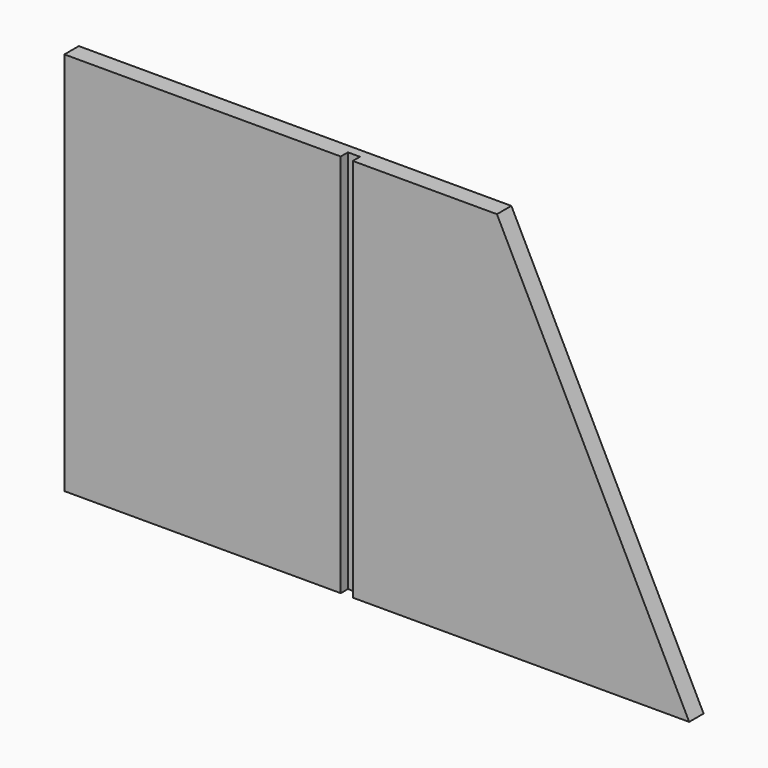
from build123d import *

# Parameters (mm, degrees)
F1_DEPTH = 19.05
F2_W     = 12.7
F2_H     = 406.4
F3_DEPTH = 9.525


# Not quite as in the source:
# - a feature names something its author has since deleted; it is built from what else it names


with BuildPart() as f1:
    # F0 (on Front) → F1 (new body)
    with BuildSketch(Plane.XZ):
        Polygon((-229.6549332498, 252.4134865394), (-356.6549332498, 252.4134865394), (-686.8549332498, 252.4134865394), (-686.8549332498, -153.9865134606), (-356.6549332498, -153.9865134606), (-229.6549332498, -153.9865134606), align=None)
        Polygon((-26.4549332498, -153.9865134606), (-229.6549332498, 252.4134865394), (-229.6549332498, -153.9865134606), align=None)
    extrude(amount=F1_DEPTH)

    # F2 (on face) → F3 (cut)
    with BuildSketch(Plane.XZ.offset(19.05)):
        with Locations((-388.4049332498, 49.2134865394)):
            Rectangle(F2_W, F2_H)
    extrude(amount=-F3_DEPTH, mode=Mode.SUBTRACT)


solid = f1.part
